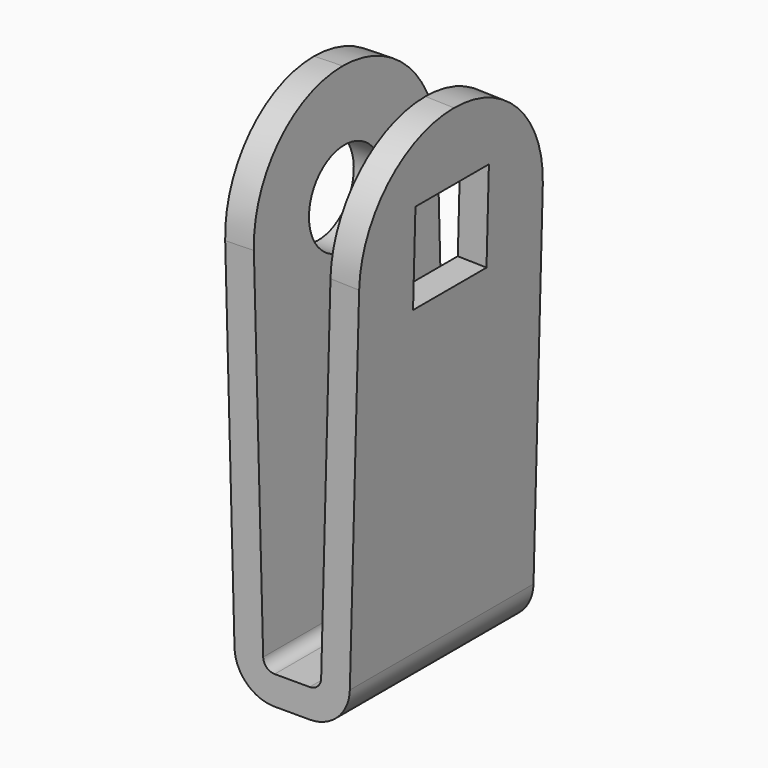
from build123d import *

# Parameters (mm, degrees)
F1_DEPTH      = 12.7
F1_DEPTH_BACK = 12.7
F2_W          = 10.16
F2_H          = 10.16
F3_DEPTH      = 3.175
F5_DEPTH      = 3.175
F6_R          = 1.27
F7_R          = 4.445
F8_D          = 10.16
F8_DEPTH      = 3.175
F8_TIP        = 3.0523719447


with BuildPart() as f1:
    # F0 (on Front) → F1 (new body, two sides)
    with BuildSketch(Plane.XZ) as f1_sk:
        Polygon((3.175, 0), (-3.175, 0), (-4.5684314445, 53.213), (-7.7423434513, 53.1298881891), (-6.2679480652, -3.175), (6.2679480652, -3.175), (7.7423434513, 53.1298881891), (4.5684314445, 53.213), align=None)
    extrude(amount=F1_DEPTH)
    extrude(f1_sk.sketch, amount=-F1_DEPTH_BACK)

    # F2 (on face) → F3 (cut, through all)
    with BuildSketch(Plane(origin=(6.3467363932, 0, -0.1661951414), x_dir=(0, 1, 0), z_dir=(0.999657325, 0, -0.0261769483))):
        with BuildLine():
            ThreePointArc((-12.7, 40.6143528277), (-8.9802561276, 49.5946089422), (-1.86e-08, 53.3143528277))
            Line((-1.86e-08, 53.3143528277), (-12.7, 53.3143528277))
            Line((-12.7, 53.3143528277), (-12.7, 40.6143528277))
        make_face()
        with BuildLine():
            ThreePointArc((-1.86e-08, 53.3143528277), (8.9802561145, 49.5946089553), (12.7, 40.6143528277))
            Line((12.7, 40.6143528277), (12.7, 53.3143528277))
            Line((12.7, 53.3143528277), (-1.86e-08, 53.3143528277))
        make_face()
        with Locations((0, 40.6143528277)):
            Rectangle(F2_W, F2_H)
    extrude(amount=-F3_DEPTH, mode=Mode.SUBTRACT)

    # F4 (on face) → F5 (cut, through all)
    with BuildSketch(Plane(origin=(-6.3467363932, 0, -0.1661951414), x_dir=(0, -1, 0), z_dir=(-0.999657325, 0, -0.0261769483))):
        with BuildLine():
            ThreePointArc((-12.7, 40.6143528277), (-8.9802561029, 49.594608967), (5.15e-08, 53.3143528277))
            Line((5.15e-08, 53.3143528277), (-12.7, 53.3143528277))
            Line((-12.7, 53.3143528277), (-12.7, 40.6143528277))
        make_face()
        with BuildLine():
            ThreePointArc((5.15e-08, 53.3143528277), (8.9802561393, 49.5946089305), (12.7, 40.6143528277))
            Line((12.7, 40.6143528277), (12.7, 53.3143528277))
            Line((12.7, 53.3143528277), (5.15e-08, 53.3143528277))
        make_face()
    extrude(amount=-F5_DEPTH, mode=Mode.SUBTRACT)

    # F6
    f6_edges = [f1.edges().sort_by_distance(p)[0] for p in [
        (3.175, 0, 0),
        (-3.175, 0, 0),
    ]]
    fillet(f6_edges, radius=F6_R)

    # F7
    f7_edges = [f1.edges().sort_by_distance(p)[0] for p in [
        (6.267948, 0, -3.175),
        (-6.267948, 0, -3.175),
    ]]
    fillet(f7_edges, radius=F7_R)

    # F8
    with Locations(Plane(origin=(-6.3467363932, 0, -0.1661951414), x_dir=(0, -1, 0), z_dir=(-0.999657325, 0, -0.0261769483))):
        with Locations((0, 40.6143528277)):
            Hole(F8_D / 2, depth=F8_DEPTH)
            with Locations((0, 0, -(F8_DEPTH + F8_TIP / 2))):  # 118° drill point
                Cone(0, F8_D / 2, F8_TIP, mode=Mode.SUBTRACT)


solid = f1.part
